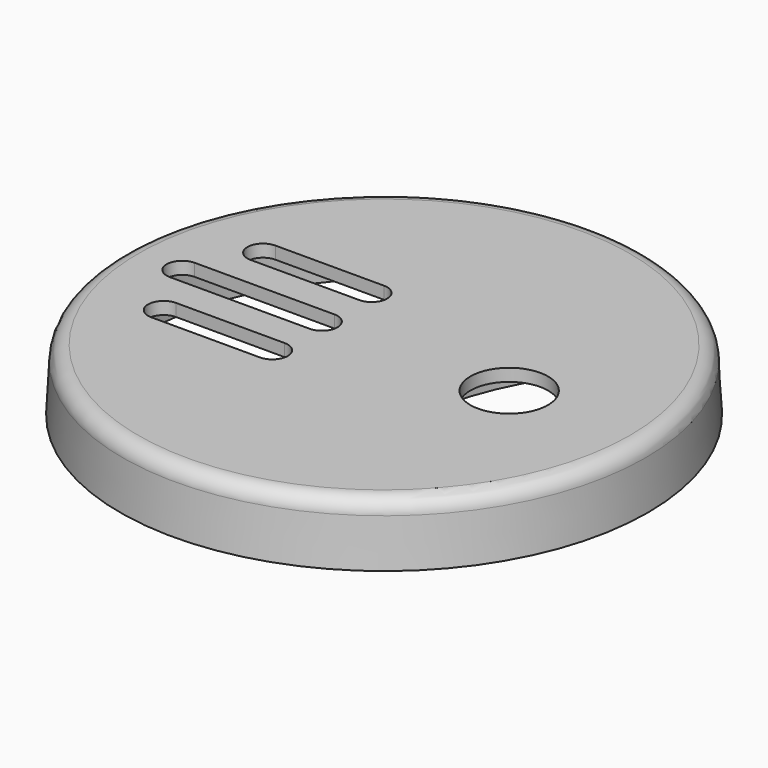
from build123d import *

# Parameters (mm, degrees)
F0_R      = 34
F1_DEPTH  = 8
F1_TAPER  = 3
F3_DEPTH  = 6.4
F3_TAPER  = 3
F5_DEPTH  = 0.8
F5_TAPER  = 3
F6_R      = 2
F8_D      = 10
F10_DEPTH = 8.8010001
F12_DEPTH = 8.8010001


with BuildPart() as f1:
    # F0 (on Top) → F1 (new body)
    with BuildSketch(Plane.XY):
        Circle(F0_R)
    extrude(amount=F1_DEPTH, taper=F1_TAPER)

    # F2 (on face) → F3 (cut)
    with BuildSketch(Plane(origin=(0, 0, 0), x_dir=(1, 0, 0), z_dir=(0, 0, -1))):
        with BuildLine():
            ThreePointArc((-12.8411571335, 24.1811270559), (-16.0020129755, 25.4015270201), (-19.2152025489, 24.3264463291))
            ThreePointArc((-19.2152025489, 24.3264463291), (-31, 0), (-19.2152025489, -24.3264463291))
            ThreePointArc((-19.2152025489, -24.3264463291), (-16.0020129755, -25.4015270201), (-12.8411571335, -24.1811270559))
            ThreePointArc((-12.8411571335, -24.1811270559), (-1.8, 0), (-12.8411571335, 24.1811270559))
        make_face()
        with BuildLine():
            ThreePointArc((12.8411571335, 24.1811270559), (1.8, 0), (12.8411571335, -24.1811270559))
            ThreePointArc((12.8411571335, -24.1811270559), (16.0020129755, -25.4015270201), (19.2152025489, -24.3264463291))
            ThreePointArc((19.2152025489, -24.3264463291), (31, 0), (19.2152025489, 24.3264463291))
            ThreePointArc((19.2152025489, 24.3264463291), (16.0020129755, 25.4015270201), (12.8411571335, 24.1811270559))
        make_face()
    extrude(amount=-F3_DEPTH, taper=F3_TAPER, mode=Mode.SUBTRACT)

    # F4 (on face) → F5 (join)
    with BuildSketch(Plane(origin=(0, 0, 0), x_dir=(1, 0, 0), z_dir=(0, 0, -1))):
        with BuildLine():
            ThreePointArc((-12.1861932939, -24.9367872764), (-0.8, 0), (-12.1861932939, 24.9367872764))
            ThreePointArc((-12.1861932939, 24.9367872764), (-15.9792203044, 26.4012672334), (-19.8350477924, 25.1111704043))
            ThreePointArc((-19.8350477924, 25.1111704043), (-32, 0), (-19.8350477924, -25.1111704043))
            ThreePointArc((-19.8350477924, -25.1111704043), (-15.9792203044, -26.4012672334), (-12.1861932939, -24.9367872764))
        make_face()
        with BuildLine():
            ThreePointArc((-19.2152025489, -24.3264463291), (-31, 0), (-19.2152025489, 24.3264463291))
            ThreePointArc((-19.2152025489, 24.3264463291), (-16.0020129755, 25.4015270201), (-12.8411571335, 24.1811270559))
            ThreePointArc((-12.8411571335, 24.1811270559), (-1.8, 0), (-12.8411571335, -24.1811270559))
            ThreePointArc((-12.8411571335, -24.1811270559), (-16.0020129755, -25.4015270201), (-19.2152025489, -24.3264463291))
        make_face(mode=Mode.SUBTRACT)
        with BuildLine():
            ThreePointArc((19.8350477924, -25.1111704043), (32, 0), (19.8350477924, 25.1111704043))
            ThreePointArc((19.8350477924, 25.1111704043), (15.9792203044, 26.4012672334), (12.1861932939, 24.9367872764))
            ThreePointArc((12.1861932939, 24.9367872764), (0.8, 0), (12.1861932939, -24.9367872764))
            ThreePointArc((12.1861932939, -24.9367872764), (15.9792203044, -26.4012672334), (19.8350477924, -25.1111704043))
        make_face()
        with BuildLine():
            ThreePointArc((12.8411571335, 24.1811270559), (16.0020129755, 25.4015270201), (19.2152025489, 24.3264463291))
            ThreePointArc((19.2152025489, 24.3264463291), (31, 0), (19.2152025489, -24.3264463291))
            ThreePointArc((19.2152025489, -24.3264463291), (16.0020129755, -25.4015270201), (12.8411571335, -24.1811270559))
            ThreePointArc((12.8411571335, -24.1811270559), (1.8, 0), (12.8411571335, 24.1811270559))
        make_face(mode=Mode.SUBTRACT)
    extrude(amount=F5_DEPTH, taper=F5_TAPER)

    # F6
    f6_edges = [f1.edges().sort_by_distance(p)[0] for p in [
        (-33.580738, 0, 8),
        (-30.66459, 0, 6.4),
        (2.13541, 0, 6.4),
    ]]
    fillet(f6_edges, radius=F6_R)

    # F8 (through all)
    with Locations(Plane.XY.offset(8)):
        with Locations((16.1159763314, 0)):
            Hole(F8_D / 2)

    # F9 (on face) → F10 (cut, through all)
    with BuildSketch(Plane.XY.offset(8)):
        with BuildLine():
            Line((-26, -2), (-8, -2))
            ThreePointArc((-8, -2), (-6, 0), (-8, 2))
            Line((-8, 2), (-26, 2))
            ThreePointArc((-26, 2), (-28, 0), (-26, -2))
        make_face()
    extrude(amount=-F10_DEPTH, mode=Mode.SUBTRACT)

    # F11 (on face) → F12 (cut, through all)
    with BuildSketch(Plane.XY.offset(8)):
        with BuildLine():
            Line((-22, 6), (-8, 6))
            ThreePointArc((-8, 6), (-6, 8), (-8, 10))
            Line((-8, 10), (-22, 10))
            ThreePointArc((-22, 10), (-24, 8), (-22, 6))
        make_face()
        with BuildLine():
            ThreePointArc((-8, -10), (-6, -8), (-8, -6))
            Line((-8, -6), (-22, -6))
            ThreePointArc((-22, -6), (-24, -8), (-22, -10))
            Line((-22, -10), (-8, -10))
        make_face()
    extrude(amount=-F12_DEPTH, mode=Mode.SUBTRACT)


solid = f1.part
